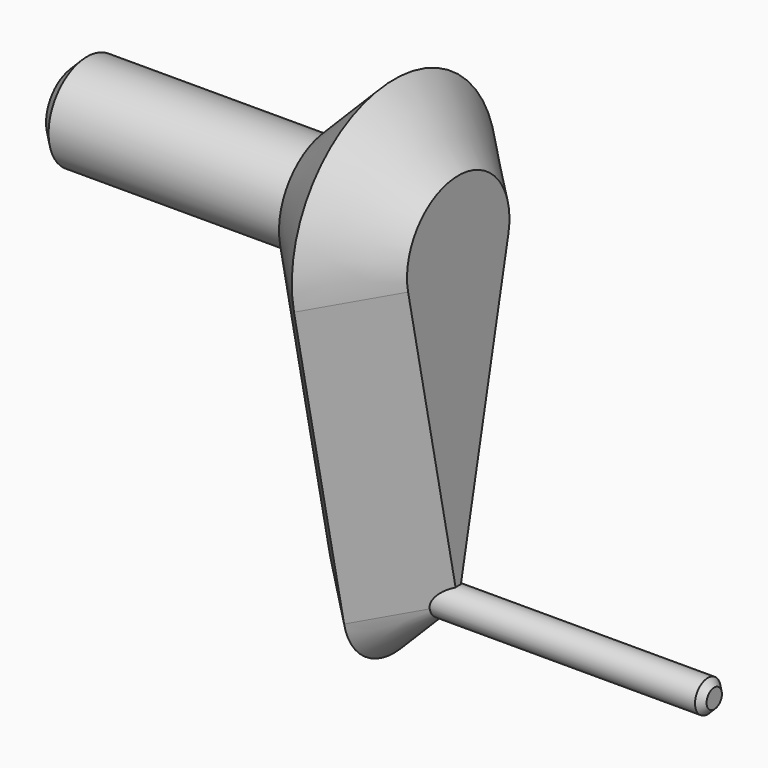
from build123d import *

# Parameters (mm, degrees)
F0_R         = 3.75
F0_R_2       = 1.25
F1_DEPTH     = 10
F2_DEPTH     = 20
F3_DEPTH     = 30
F4_T1_DEPTH  = 23.936451485
F4_T3_DEPTH  = 23.936451485
F4_T8_DEPTH  = 23.936451485
F4_S9_R      = 1.25
F4_T10_DEPTH = 15
F4_T14_ANGLE = 156.4026846179
F4_S15_R     = 1.25
F4_T16_DEPTH = 8
F4_T18_ANGLE = 203.5973153821
F4_T22_DEPTH = 23.936451485
F4_S23_R     = 1.25
F4_T24_DEPTH = 15
F4_T26_ANGLE = 156.4026846179
F4_T28_ANGLE = 203.5973153821
F5_SIZE      = 1
F6_SIZE      = 0.5


# Not quite as in the source:
# - a fillet or chamfer that OpenCascade refuses, or shapes differently, is made with other operations: its cross-section is extruded or revolved along the edge and cut away or added


with BuildPart() as f1:
    # F0 (on Right) → F1 (new body)
    with BuildSketch(Plane.YZ):
        with BuildLine():
            ThreePointArc((3.6919470815, 19.2276737533), (3.8502654993, 20.2445960951), (3.9032252878, 21.2724049449))
            ThreePointArc((3.9032252878, 21.2724049449), (-7.124583562, 31.2194451563), (-15.8854965059, 19.2276737533))
            ThreePointArc((-15.8854965059, 19.2276737533), (-6.0967747122, 11.2724049449), (3.6919470815, 19.2276737533))
        make_face()
        with Locations((-6.0967747122, 21.2724049449)):
            Circle(F0_R, mode=Mode.SUBTRACT)
        with BuildLine():
            ThreePointArc((3.6919470815, 19.2276737533), (-6.0967747122, 11.2724049449), (-15.8854965059, 19.2276737533))
            Line((-15.8854965059, 19.2276737533), (-10.991135609, -4.2030526781))
            ThreePointArc((-10.991135609, -4.2030526781), (-6.6106791371, 1.7928330234), (-1.0967747122, -3.1806870823))
            ThreePointArc((-1.0967747122, -3.1806870823), (-1.1232546065, -3.6945915072), (-1.2024138154, -4.2030526781))
            Line((-1.2024138154, -4.2030526781), (3.6919470815, 19.2276737533))
        make_face()
        with BuildLine():
            ThreePointArc((-1.0967747122, -3.1806870823), (-6.6106791371, 1.7928330234), (-10.991135609, -4.2030526781))
            ThreePointArc((-10.991135609, -4.2030526781), (-6.0967747122, -8.1806870823), (-1.2024138154, -4.2030526781))
            ThreePointArc((-1.2024138154, -4.2030526781), (-1.1232546065, -3.6945915072), (-1.0967747122, -3.1806870823))
        make_face()
        with Locations((-6.0967747122, -3.1806870823)):
            Circle(F0_R_2, mode=Mode.SUBTRACT)
        with Locations((-6.0967747122, 21.2724049449)):
            Circle(F0_R)
        with Locations((-6.0967747122, -3.1806870823)):
            Circle(F0_R_2)
    extrude(amount=F1_DEPTH)

    # F0 (on Right) → F2 (join)
    with BuildSketch(Plane.YZ):
        with Locations((-6.0967747122, 21.2724049449)):
            Circle(F0_R)
    extrude(amount=-F2_DEPTH)

    # F0 (on Right) → F3 (join)
    with BuildSketch(Plane.YZ):
        with Locations((-6.0967747122, -3.1806870823)):
            Circle(F0_R_2)
    extrude(amount=F3_DEPTH)

    # F4: chamfer of 5 on 2 edges, made by hand

    # F4_s2 → F4_t1 (cut)
    with BuildSketch(Plane(origin=(0, -0.8915258311, -4.2679929606), x_dir=(1, 0, 0), z_dir=(0, 0.2044731192, 0.9788721794))):
        Polygon((5, -0.3175981408), (0, -5.3175981408), (0, -0.3175981408), align=None)
    extrude(amount=F4_T1_DEPTH, mode=Mode.SUBTRACT)

    # F4_s4 → F4_t3 (cut)
    with BuildSketch(Plane(origin=(0, -4.5126383008, 21.6033095513), x_dir=(1, 0, 0), z_dir=(0, 0.2044731192, -0.9788721794))):
        Polygon((5, 11.6183281585), (0, 6.6183281585), (0, 11.6183281585), align=None)
    extrude(amount=F4_T3_DEPTH, mode=Mode.SUBTRACT)


with BuildPart() as f4_tool6:
    # F4_s7 → F4_t8 (new body)
    with BuildSketch(Plane(origin=(0, -0.8915258311, -4.2679929606), x_dir=(1, 0, 0), z_dir=(0, 0.2044731192, 0.9788721794))):
        Polygon((5, -0.3175981408), (10, -5.3175981408), (10, -0.3175981408), align=None)
    extrude(amount=F4_T8_DEPTH)

    # F4_s9 → F4_t10 (cut, symmetric)
    with BuildSketch(Plane.YZ.offset(7.5)):
        with Locations((-6.0967747122, -3.1806870823)):
            Circle(F4_S9_R)
    extrude(amount=F4_T10_DEPTH, both=True, mode=Mode.SUBTRACT)


with BuildPart() as f1_1:
    add(f1.part)

    # F4_t5: cut F4_tool6
    add(f4_tool6.part, mode=Mode.SUBTRACT)


with BuildPart() as f4_tool12:
    # F4_s13 → F4_t14 (revolve)
    with BuildSketch(Plane(origin=(0, 0.381722596, -1.8274168801), x_dir=(1, 0, 0), z_dir=(0, -0.2044731192, 0.9788721794))):
        Polygon((10, -6.6183281585), (5, -11.6183281585), (10, -11.6183281585), align=None)
    revolve(axis=Axis((10, -6.0967747122, -3.1806870823), (1, 0, 0)), revolution_arc=F4_T14_ANGLE)

    # F4_s15 → F4_t16 (cut, symmetric)
    with BuildSketch(Plane.YZ.offset(7.5)):
        with Locations((-6.0967747122, -3.1806870823)):
            Circle(F4_S15_R)
    extrude(amount=F4_T16_DEPTH, both=True, mode=Mode.SUBTRACT)


with BuildPart() as f1_2:
    add(f1_1.part)

    # F4_t11: cut F4_tool12
    add(f4_tool12.part, mode=Mode.SUBTRACT)

    # F4_s17 → F4_t18 (revolve, cut)
    with BuildSketch(Plane(origin=(0, 4.0028350658, 19.1627334708), x_dir=(1, 0, 0), z_dir=(0, -0.2044731192, -0.9788721794))):
        Polygon((5, 0.3175981408), (10, 5.3175981408), (10, 0.3175981408), align=None)
    revolve(axis=Axis((10, -6.0967747122, 21.2724049449), (1, 0, 0)), revolution_arc=F4_T18_ANGLE, mode=Mode.SUBTRACT)


with BuildPart() as f4_tool20:
    # F4_s21 → F4_t22 (new body)
    with BuildSketch(Plane(origin=(0, -4.5126383008, 21.6033095513), x_dir=(1, 0, 0), z_dir=(0, 0.2044731192, -0.9788721794))):
        Polygon((5, 11.6183281585), (10, 6.6183281585), (10, 11.6183281585), align=None)
    extrude(amount=F4_T22_DEPTH)

    # F4_s23 → F4_t24 (cut, symmetric)
    with BuildSketch(Plane.YZ.offset(7.5)):
        with Locations((-6.0967747122, -3.1806870823)):
            Circle(F4_S23_R)
    extrude(amount=F4_T24_DEPTH, both=True, mode=Mode.SUBTRACT)


with BuildPart() as f1_3:
    add(f1_2.part)

    # F4_t19: cut F4_tool20
    add(f4_tool20.part, mode=Mode.SUBTRACT)

    # F4_s25 → F4_t26 (revolve, cut)
    with BuildSketch(Plane(origin=(0, 0.381722596, -1.8274168801), x_dir=(1, 0, 0), z_dir=(0, -0.2044731192, 0.9788721794))):
        Polygon((0, -6.6183281585), (5, -11.6183281585), (0, -11.6183281585), align=None)
    revolve(axis=Axis((0, -6.0967747122, -3.1806870823), (1, 0, 0)), revolution_arc=F4_T26_ANGLE, mode=Mode.SUBTRACT)

    # F4_s27 → F4_t28 (revolve, cut)
    with BuildSketch(Plane(origin=(0, 4.0028350658, 19.1627334708), x_dir=(1, 0, 0), z_dir=(0, -0.2044731192, -0.9788721794))):
        Polygon((5, 0.3175981408), (0, 5.3175981408), (0, 0.3175981408), align=None)
    revolve(axis=Axis((0, -6.0967747122, 21.2724049449), (1, 0, 0)), revolution_arc=F4_T28_ANGLE, mode=Mode.SUBTRACT)

    # F5
    f5_edges = [f1_3.edges().sort_by_distance(p)[0] for p in [
        (-20, -9.846775, 21.272405),
    ]]
    chamfer(f5_edges, length=F5_SIZE)

    # F6
    f6_edges = [f1_3.edges().sort_by_distance(p)[0] for p in [
        (30, -7.346775, -3.180687),
    ]]
    chamfer(f6_edges, length=F6_SIZE)


solid = f1_3.part
